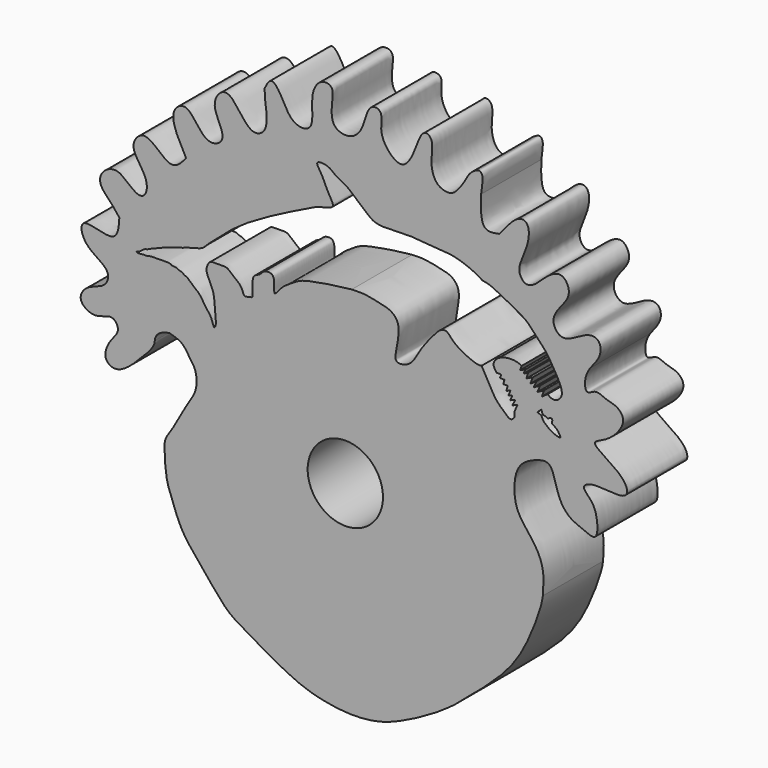
from build123d import *

# Parameters (mm, degrees)
F1_DEPTH  = 6.35
F3_DEPTH  = 25.4
F5_DEPTH  = 25.4
F6_R      = 3.175
F7_DEPTH  = 25.4
F8_DEPTH  = 6.35
F10_DEPTH = 25.4


with BuildPart() as f1:
    # F0 (on Front) → F1 (new body)
    with BuildSketch(Plane.XZ):
        with BuildLine():
            add(Edge.make_bspline(
                [(10.9984036535, 24.0315832198), (11.2508201386, 23.8778308248), (11.5032366237, 23.7240784298), (11.5215126425, 23.4777014703)],
                knots=[0, 0, 0, 0, 0.0447233475, 0.0447233475, 0.0447233475, 0.0447233475], degree=3))
            add(Edge.make_bspline(
                [(10.9984036535, 24.0315832198), (11.318751732, 24.2589387251), (11.9002035172, 24.6716031777), (12.4772696509, 24.5492373746), (12.7513167847, 24.476788925)],
                knots=[0, 0, 0, 0, 0.0600549328, 0.1090034566, 0.1090034566, 0.1090034566, 0.1090034566], degree=3))
            add(Edge.make_bspline(
                [(12.7513167847, 24.476788925), (12.7801536971, 24.4691654569), (13.1432187191, 24.3713046181), (13.9041914038, 24.1543272236), (14.4865013027, 23.118412087), (15.0212391704, 22.4815104313), (15.1483784966, 20.9912222479), (14.3534367186, 19.8288905944), (13.7773894226, 18.8194596912), (13.1463892826, 17.6016964054), (12.3275103111, 16.5516353367), (12.33673354, 15.5224584087), (12.4614385645, 13.4803711032), (12.9391618875, 12.3662133846), (13.3935402384, 11.0178879135), (13.885287327, 10.0483936843), (14.2166576245, 9.5778162211), (14.3705829978, 9.3592274934)],
                knots=[0.1090034566, 0.1090034566, 0.1090034566, 0.1090034566, 0.1141541191, 0.1734825658, 0.2342293124, 0.2866985313, 0.3540034981, 0.4216578627, 0.4838023186, 0.5515034671, 0.6159797954, 0.6739052407, 0.7551671162, 0.8199016797, 0.887742666, 0.9478551573, 1, 1, 1, 1], degree=3))
            add(Edge.make_bspline(
                [(14.3705829978, 9.3592274934), (14.7206651853, 8.9162577102), (15.4412953386, 8.0044221636), (16.7099442924, 6.5073513391), (17.7815135431, 5.221403597), (19.802190403, 4.1080383003), (22.0570488159, 2.7795203295), (24.6499909887, 1.5346825958), (28.0004167304, 1.0133030815), (30.4911131278, 1.2899704351), (32.5358810979, 2.0983522438), (35.0221117989, 3.4149839779), (36.2013376915, 4.264379538), (36.7506444454, 4.6600447968)],
                knots=[0, 0, 0, 0, 0.0782058444, 0.1609835967, 0.2374772319, 0.3265742131, 0.4230092715, 0.5241503873, 0.6331121598, 0.7261758396, 0.8140180236, 0.9133659154, 1, 1, 1, 1], degree=3))
            add(Edge.make_bspline(
                [(36.7506444454, 4.6600447968), (38.0482118698, 5.7380044032), (40.4681398718, 7.7483697897), (42.6588108138, 10.3810181384), (44.0911971273, 14.1984339335), (44.2071973729, 14.954150476), (44.2453101277, 15.2024468407)],
                knots=[0, 0, 0, 0, 0.3118653648, 0.5816204345, 0.8625382411, 1, 1, 1, 1], degree=3))
            add(Edge.make_bspline(
                [(44.2453101277, 15.2024468407), (44.2938227776, 15.848400886), (44.3896532958, 17.1244002587), (43.6653685125, 18.8179219808), (42.1824281003, 20.4121601043), (41.7448299587, 22.0053036238), (41.9549170872, 24.3004416385), (43.5573707454, 25.1201218431), (44.8828418523, 25.4189210069), (45.2842380478, 24.0145128143), (45.7035890114, 22.5708511362), (46.5789159349, 21.6207741355), (47.6415206601, 21.2667344741), (48.8901196768, 20.6378885116), (48.8646803505, 22.5006482664), (48.45281122, 23.5890104482), (47.4324727249, 24.3843013724), (48.2991800009, 24.9299049673), (49.7655119556, 24.745912619), (51.4805558413, 24.7166370614), (51.2824255696, 26.0405470322), (49.613217734, 27.141164769), (48.2215617536, 28.0385485724), (49.6100830633, 28.4546279683), (50.7055587208, 29.4428489996), (51.203797615, 30.5543020473), (50.4972683382, 31.3694856565), (49.523918889, 31.4773590202), (48.7198259044, 32.0094415516), (47.8360516345, 31.2174357433), (47.7324347795, 32.5701272714), (48.0509651737, 33.1047449245), (48.2145175338, 33.3792492747)],
                knots=[0, 0, 0, 0, 0.040744066, 0.0804846769, 0.1234849874, 0.1615884455, 0.2044023143, 0.2429972637, 0.2738845866, 0.3065024407, 0.3436012027, 0.3761355316, 0.4085263524, 0.4373910774, 0.4719923049, 0.5062540019, 0.5354026429, 0.5590121233, 0.5967931375, 0.6319390032, 0.6593392118, 0.7029962174, 0.7347840934, 0.7637562386, 0.8011345948, 0.8317135686, 0.8595523187, 0.8888743382, 0.9167130857, 0.9421066461, 0.9702741251, 1, 1, 1, 1], degree=3))
            add(Edge.make_bspline(
                [(48.2145175338, 33.3792492747), (48.5950355002, 33.8439156617), (49.2587706884, 34.6544304313), (49.0258880789, 35.8281927213), (47.8540536179, 35.9750774666), (45.8946501082, 34.3557167277), (44.8208041616, 35.9630519047), (45.7909681384, 37.2143462577), (46.7270923619, 38.3660487916), (45.9004450462, 39.8804900002), (44.462754299, 39.0181229163), (43.6562779713, 38.05713357), (42.7278190322, 37.7260580899), (42.1458451865, 38.5754480959), (42.3827930851, 39.4928006532), (42.9237980131, 40.5832499857), (43.1672501036, 41.9085122108), (42.8104534524, 42.6456809415), (41.9271647427, 42.5728848132), (41.1081073815, 41.5433021848), (40.5772328377, 40.8759750426)],
                knots=[0, 0, 0, 0, 0.0649588079, 0.1133072558, 0.162889424, 0.2379143585, 0.2939815841, 0.355441398, 0.4157416364, 0.4709310898, 0.5298717766, 0.5887591138, 0.6338079166, 0.679457886, 0.7275283161, 0.7843150664, 0.8428561205, 0.8840239325, 0.9248297557, 1, 1, 1, 1], degree=3))
            add(Edge.make_bspline(
                [(39.0425574679, 43.3239779902), (39.041356185, 43.2750910809), (39.0219364766, 42.5343034751), (38.9455255975, 40.5484904636), (40.0875605821, 40.77769754), (40.5772328377, 40.8759750426)],
                knots=[0.922393852, 0.922393852, 0.922393852, 0.922393852, 0.9255178455, 0.9680641617, 1, 1, 1, 1], degree=3))
            add(Edge.make_bspline(
                [(37.5906317725, 43.7307091179), (37.837040982, 44.0878360909), (38.2680272592, 44.6707408411), (38.9849891485, 45.0931421059), (39.0542753062, 44.2835962885), (39.0533749724, 43.7642026309), (39.0425574679, 43.3239779902)],
                knots=[0.8216596087, 0.8216596087, 0.8216596087, 0.8216596087, 0.8509906652, 0.8729404344, 0.8942624168, 0.922393852, 0.922393852, 0.922393852, 0.922393852], degree=3))
            add(Edge.make_bspline(
                [(20.7812990993, 45.2349446714), (20.9598079298, 45.5940884592), (21.3279572872, 46.3347720119), (22.249821537, 45.1800137174), (22.9935969334, 43.2743045581), (25.1488502819, 43.2665919302), (24.5153462292, 46.05875701), (25.4553091101, 47.4888604199), (26.6873108255, 47.2876915045), (26.3981434507, 45.832663308), (26.4326586416, 44.1475738694), (28.033955093, 43.8270222859), (29.0048714578, 44.7100760367), (29.2810737014, 45.9686995054), (29.7673820709, 47.0106125091), (30.7919294346, 46.7608773347), (30.4737375786, 45.4274062089), (30.9768926389, 44.0748322152), (32.5368669527, 42.8415889335), (33.5078035863, 44.7935011377), (33.9248822803, 46.1667164525), (34.4543244348, 46.441199242), (34.9775884722, 46.0257106289), (34.8859088958, 44.9334895069), (34.8042115189, 44.1708427609), (35.1252581337, 42.7624795784), (36.6346449921, 42.3082232141), (37.2318305413, 43.2058580932), (37.5522842498, 43.6751311032), (37.5906317725, 43.7307091179)],
                knots=[0, 0, 0, 0, 0.0277218275, 0.0571723705, 0.0983426517, 0.1308747904, 0.1751695472, 0.2104503073, 0.2359276255, 0.2684453241, 0.3038767035, 0.3359700253, 0.3670382979, 0.3999783047, 0.4285856537, 0.4517548965, 0.482396946, 0.5175640575, 0.5519099854, 0.5898501594, 0.6248167325, 0.6437016849, 0.6642895518, 0.6932428536, 0.7192839991, 0.751939533, 0.7835122944, 0.8170949524, 0.8216596087, 0.8216596087, 0.8216596087, 0.8216596087], degree=3))
            add(Edge.make_bspline(
                [(14.1616091132, 37.9098691046), (13.5322036704, 39.0585651197), (12.5165881256, 40.9121136432), (14.415081949, 42.2942809419), (15.6801738753, 39.2181703105), (17.8891113724, 40.288290195), (16.1164787578, 42.4584838578), (17.1043617929, 43.9976160978), (18.2133555313, 43.7714508614), (19.5101751542, 41.2574608503), (21.2098070485, 42.0889312218), (20.7967934332, 44.364971779), (20.7856516925, 44.9905561021), (20.7812990993, 45.2349446714)],
                knots=[0, 0, 0, 0, 0.1255875684, 0.2026494815, 0.3148208465, 0.394753195, 0.4994852093, 0.581932278, 0.6470220286, 0.7573364877, 0.8326463523, 0.9346222132, 1, 1, 1, 1], degree=3))
            add(Edge.make_bspline(
                [(8.5367122665, 31.6628292203), (8.3127892358, 31.9583180313), (7.8541426883, 32.563547974), (6.8806160847, 33.4557075972), (6.8883368651, 34.3315498499), (7.47477818, 34.9861300171), (8.3402060898, 35.1611632264), (8.970020513, 34.7214135391), (9.6560863557, 34.1403407566), (10.1718011229, 33.8172376038), (10.7815639847, 33.9576662574), (10.978297702, 35.0741741128), (10.2142510997, 36.2695531421), (9.4105325611, 37.4621624953), (10.7801226417, 39.1527841943), (12.8559031413, 36.3266719936), (13.7632400269, 37.4268378556), (14.1616091132, 37.9098691046)],
                knots=[0, 0, 0, 0, 0.0694766566, 0.1423043829, 0.198764402, 0.2572227337, 0.3150056147, 0.3706419002, 0.4324868971, 0.4819124791, 0.5268043346, 0.5899069271, 0.6677982109, 0.7421643789, 0.816159908, 0.9192844349, 1, 1, 1, 1], degree=3))
            add(Edge.make_bspline(
                [(11.5215126425, 23.4777014703), (11.5519824112, 23.0669419365), (10.2609372621, 21.6762525704), (8.4228613972, 19.9629948924), (7.0758637078, 20.791261283), (7.7048728638, 22.3612173674), (8.6771579986, 23.1802967965), (7.9435187696, 24.4141861888), (6.5366962855, 23.4032665751), (4.921446276, 24.3963742293), (5.7309585025, 25.8129083909), (7.4360032754, 26.0087969672), (7.8559307485, 27.6450981333), (5.5063417726, 28.4696216823), (5.0165874684, 31.0102223234), (8.3946531142, 29.35366443), (8.4920119608, 30.9362278683), (8.5367122665, 31.6628292203)],
                knots=[0.0447233475, 0.0447233475, 0.0447233475, 0.0447233475, 0.1192860883, 0.1999034705, 0.251345599, 0.3134883632, 0.3693216082, 0.417594106, 0.4791297169, 0.5399528379, 0.5960189727, 0.661036052, 0.7147344751, 0.7926602543, 0.8538783164, 0.9329112437, 1, 1, 1, 1], degree=3))
        make_face()
        with BuildLine():
            add(Edge.make_bspline(
                [(37.5906317725, 43.7307091179), (37.6583476274, 43.8577441648), (37.7894200704, 44.1020132691), (37.9701475696, 44.4125750304), (38.2660625267, 44.7503024581), (38.617932892, 44.9570790944), (38.9662554933, 45.071039684), (39.1943363106, 44.7057833587), (39.1494306301, 44.1431294325), (39.0811155736, 43.6150886764), (39.0425574679, 43.3239779902)],
                knots=[0, 0, 0, 0, 0.1208224911, 0.2327121383, 0.3564976038, 0.4773631849, 0.5804917461, 0.6891217609, 0.828579593, 1, 1, 1, 1], degree=3))
            add(Edge.make_bspline(
                [(37.5906317725, 43.7307091179), (37.837040982, 44.0878360909), (38.2680272592, 44.6707408411), (38.9849891485, 45.0931421059), (39.0542753062, 44.2835962885), (39.0533749724, 43.7642026309), (39.0425574679, 43.3239779902)],
                knots=[0.8216596087, 0.8216596087, 0.8216596087, 0.8216596087, 0.8509906652, 0.8729404344, 0.8942624168, 0.922393852, 0.922393852, 0.922393852, 0.922393852], degree=3))
        make_face()
    extrude(amount=F1_DEPTH)

    # F2 (on face) → F3 (cut)
    with BuildSketch(Plane.XZ.offset(6.35)):
        with BuildLine():
            add(Edge.make_bspline(
                [(10.9213702381, 30.0800928582), (11.0621325147, 30.1711970051), (11.4478540925, 30.3014983827), (12.6817518677, 30.859944003), (13.7072983183, 31.0710903888), (14.3208772689, 31.3579432612), (15.564229897, 31.570259495), (16.0136899008, 32.1813542456), (17.049722233, 32.9854347042), (18.3746171419, 34.2826629705), (21.6392706703, 36.1544500181), (23.5400043531, 37.0799669008), (24.4557429105, 37.5258624554)],
                knots=[0, 0, 0, 0, 0.0624681448, 0.1605025237, 0.2463917171, 0.3163794584, 0.4075323766, 0.479568724, 0.5724130102, 0.6875313423, 0.8499041867, 1, 1, 1, 1], degree=3))
            add(Edge.make_bspline(
                [(10.9213702381, 30.0800928582), (10.8182955843, 30.060403049), (10.6160561956, 30.0217703219), (10.4055464041, 29.8084417721), (10.1990968304, 29.6832850534), (9.8446723952, 29.5882293745), (10.2918300979, 29.5188273702), (10.5647671852, 29.602504464), (10.8901845547, 29.5492359826), (11.1801832433, 29.6758527354), (11.4710576538, 29.6348812436), (11.8361269725, 29.6727692435), (12.0701749285, 29.6638357746), (12.3013535347, 29.6671041387), (12.4604577777, 29.6625090516), (12.642664173, 29.6801227261), (12.9175606543, 29.6119395683), (12.9813179246, 29.5210420262), (13.2639078187, 29.5491884683), (13.4567806443, 29.4620166023), (13.6101856596, 29.3803257023), (13.8016463931, 29.3527375965), (13.9617442467, 29.2057757716), (14.262979255, 29.0863052722), (14.33562829, 29.011155294), (14.5563019527, 28.8115816148), (14.7331123665, 28.6495022445), (14.9650783705, 28.4431672158), (15.2472798972, 28.2700092196), (15.6300765823, 27.7063340855), (15.9140629032, 27.229935805), (16.3288629431, 26.8078143592), (16.4898288734, 25.9640936837), (16.7113330192, 26.3395278682), (16.6440586968, 26.8944387045), (16.6245707773, 27.4260731323), (16.5646216855, 27.9561127995), (16.4922967389, 28.7242841841), (16.2171922513, 29.228497163), (16.0502440225, 29.60383452), (15.8498940382, 30.0972798293), (15.9242114176, 30.4715311828), (16.1301596613, 30.8951597944), (16.5022073659, 30.9337885236), (16.8598977355, 30.925444839), (17.2230428243, 30.9204375143), (17.6123193522, 30.9510625485), (18.0208450694, 30.5484633884), (18.4124488922, 30.2275658458), (18.8579724683, 29.9205017207), (19.0273748777, 29.2065876594), (19.2289940195, 29.3060397701), (19.3648556717, 29.2536751868), (19.5658344037, 29.4027199569), (19.6758211775, 29.3466416068), (19.7907481863, 29.4687530524), (19.7426666547, 29.679034281), (19.7359344634, 30.6677243546), (19.9019423697, 31.1236509256), (20.4493921261, 31.280142146), (20.6617274484, 31.6822365954), (21.4582760395, 31.7883774062), (21.6455719921, 31.155598957), (21.5160445037, 29.953434889), (22.1189328434, 30.89800932), (22.8009179427, 31.3425690523), (23.5862555743, 31.8845985236), (24.3790029645, 32.1394947537), (25.5496803949, 32.34015209), (26.4432119532, 32.5062561098), (27.304817882, 32.5973834381), (27.8581011731, 32.6687042567), (28.1333383173, 32.7041836191)],
                knots=[0, 0, 0, 0, 0.0124943974, 0.0245148463, 0.0364334491, 0.0467508795, 0.058726404, 0.0716998514, 0.0842925533, 0.0966964264, 0.1089343296, 0.1225436985, 0.1336494248, 0.144351145, 0.1532555432, 0.163099707, 0.1747943426, 0.1819615768, 0.1934698517, 0.2040261437, 0.2133410066, 0.2229314519, 0.2336489854, 0.2462026284, 0.2537133066, 0.2656888042, 0.277132901, 0.289381368, 0.3023902215, 0.3208309997, 0.3377388974, 0.3559011538, 0.3738992488, 0.3842692937, 0.4015763024, 0.418119285, 0.4346836826, 0.454495423, 0.4714671739, 0.4860581943, 0.5021549002, 0.5161409215, 0.5308917231, 0.5440478608, 0.5576495421, 0.5712512234, 0.5848836089, 0.6015159078, 0.6177276563, 0.6346555721, 0.6524091162, 0.6608042319, 0.6691994042, 0.6799011415, 0.6871715086, 0.6950641937, 0.7053460917, 0.7277566769, 0.7432686553, 0.7591566332, 0.7741434845, 0.7919830937, 0.8097539618, 0.8299061546, 0.8480781119, 0.8698967765, 0.8915050665, 0.9122189323, 0.9367396177, 0.958502005, 0.9793563445, 1, 1, 1, 1], degree=3))
            add(Edge.make_bspline(
                [(28.1333383173, 32.7041836191), (28.4447338183, 32.7147448415), (29.1283937094, 32.760138923), (30.4928781187, 32.4625611087), (31.4747994534, 32.2455623678), (32.1565235724, 31.4999370771), (32.059282622, 30.2460859406), (31.8173684326, 29.1896037218), (31.792310072, 28.5462210928), (32.4201594265, 28.4647743828), (33.1831286949, 28.8241096157), (33.5558384411, 29.5009799351), (34.0187523078, 30.2669265073), (34.5293868658, 30.9637754806), (35.1225494167, 31.6599302024), (35.5084483018, 32.0909391799), (36.1265305642, 32.3579699138), (36.6667314638, 31.5645481621), (37.6564672856, 30.9817736061), (38.6799457652, 30.5513126095), (38.973828395, 30.5873574143), (39.0821322799, 30.6006409228)],
                knots=[0, 0, 0, 0, 0.0569144606, 0.1245771675, 0.1817876373, 0.2355106649, 0.2987629217, 0.359895433, 0.4006617079, 0.4408969185, 0.4925680808, 0.542591235, 0.5965146494, 0.6504445858, 0.7049104477, 0.7489486043, 0.7902974011, 0.8423332006, 0.9057877046, 0.965265946, 1, 1, 1, 1], degree=3))
            add(Edge.make_bspline(
                [(39.0821322799, 30.6006409228), (39.2965137066, 30.2458058271), (39.7205354547, 29.5441861059), (40.218174815, 28.4578704854), (41.0526669064, 27.7505771838), (41.5272187519, 27.2917509414), (42.0679852633, 27.8149798012), (41.4297583603, 28.9211768264), (40.8534983099, 30.056962233), (39.8275546559, 30.9348100284), (40.5191768137, 31.8051609064), (41.7155009482, 31.9744597758), (42.5513788626, 31.7177248026), (43.7825538999, 30.8855475191), (44.5622137989, 30.3708020434), (45.1623077351, 29.8853459199), (46.2152371998, 30.5913010892), (45.1848802623, 32.3130075341), (44.5962190379, 33.3763475906), (43.6647534314, 34.2907294849), (43.0457859768, 35.0790449938), (41.9609214475, 35.7636010234), (40.9091454733, 36.2240410817), (39.9405635142, 36.8174269381), (39.3920691489, 36.9128081003), (39.140265435, 36.9565971196)],
                knots=[0, 0, 0, 0, 0.0471289622, 0.0934992279, 0.1381013781, 0.1691653891, 0.1983013447, 0.2437746361, 0.2940659419, 0.3389748368, 0.3774362068, 0.4229118573, 0.4627941098, 0.5140815647, 0.5559837663, 0.5903984763, 0.62926846, 0.6853848868, 0.734378372, 0.7815503832, 0.8241503815, 0.8714534974, 0.917581552, 0.9622845444, 1, 1, 1, 1], degree=3))
            add(Edge.make_bspline(
                [(24.4557429105, 37.5258624554), (24.7253385406, 37.6679074084), (25.269000354, 37.9543527664), (26.2041876384, 38.1068656578), (26.7222447476, 38.390498104), (26.0571499962, 39.2934646114), (25.7120527401, 40.3463293225), (25.0259646789, 41.1902198608), (25.6192781851, 41.3211522067), (26.2749340242, 41.1753665803), (26.7558685385, 40.6898514014), (27.5394779114, 40.37141568), (28.333800935, 39.7426144748), (29.3119296607, 38.8398867041), (29.9261777829, 38.3487917662), (30.5795011701, 38.2059401352), (31.5837794212, 38.2066358352), (32.438061969, 38.2621120222), (33.4591861971, 38.2772266445), (34.2594025193, 38.1616941856), (35.5273603681, 38.1006369361), (36.9245225402, 38.0116693913), (38.5905711621, 37.3317489081), (38.9903120203, 37.0589363552), (39.140265435, 36.9565971196)],
                knots=[0, 0, 0, 0, 0.0462405859, 0.0932479536, 0.12352938, 0.1694573257, 0.2239012849, 0.2673722591, 0.2966816534, 0.3360973889, 0.3752190307, 0.4184715797, 0.4672989686, 0.5228690875, 0.5647361691, 0.6030394988, 0.6506723572, 0.6959270297, 0.7435553104, 0.786874903, 0.8398639848, 0.8982460293, 0.9618293826, 1, 1, 1, 1], degree=3))
        make_face()
    extrude(amount=-F3_DEPTH, mode=Mode.SUBTRACT)

    # F4 (on face) → F5 (cut)
    with BuildSketch(Plane.XZ.offset(6.35)):
        with BuildLine():
            Line((41.6713940372, 29.2312545242), (41.334032409, 29.1238261514))
            add(Edge.make_bspline(
                [(41.4966993879, 28.8241959522), (41.4898705966, 28.8366803131), (41.4346962394, 28.9376267554), (41.3810155374, 29.0374196072), (41.334032409, 29.1238261514)],
                knots=[0.2423069379, 0.2423069379, 0.2423069379, 0.2423069379, 0.2437746361, 0.2541872492, 0.2541872492, 0.2541872492, 0.2541872492], degree=3))
            Line((41.4966993879, 28.8241959522), (41.6713940372, 29.2312545242))
        make_face()
        with BuildLine():
            Line((41.5145814011, 29.5445260139), (41.1690312073, 29.4201169181))
            add(Edge.make_bspline(
                [(41.334032409, 29.1238261514), (41.2795068463, 29.2241039661), (41.2250699584, 29.3229570106), (41.1690312073, 29.4201169181)],
                knots=[0.2541872492, 0.2541872492, 0.2541872492, 0.2541872492, 0.2662714507, 0.2662714507, 0.2662714507, 0.2662714507], degree=3))
            Line((41.334032409, 29.1238261514), (41.5145814011, 29.5445260139))
        make_face()
        with BuildLine():
            Line((41.286166143, 29.8312112658), (40.9100426519, 29.8312112658))
            add(Edge.make_bspline(
                [(41.1690312073, 29.4201169181), (41.0877859462, 29.560979837), (41.0031736736, 29.6982838928), (40.9100426519, 29.8312112658)],
                knots=[0.2662714507, 0.2662714507, 0.2662714507, 0.2662714507, 0.2837911864, 0.2837911864, 0.2837911864, 0.2837911864], degree=3))
            Line((41.1690312073, 29.4201169181), (41.286166143, 29.8312112658))
        make_face()
        with BuildLine():
            Line((41.0126723506, 30.1930415904), (40.6225825999, 30.1930415904))
            add(Edge.make_bspline(
                [(40.9100426519, 29.8312112658), (40.855424335, 29.9091688492), (40.7634152709, 30.0314018438), (40.6612602523, 30.1493652065), (40.6225825999, 30.1930415904)],
                knots=[0.2837911864, 0.2837911864, 0.2837911864, 0.2837911864, 0.2940659419, 0.3002186185, 0.3002186185, 0.3002186185, 0.3002186185], degree=3))
            Line((40.9100426519, 29.8312112658), (41.0126723506, 30.1930415904))
        make_face()
        with BuildLine():
            Line((40.7454008838, 30.4925257189), (40.3571343923, 30.4925257189))
            add(Edge.make_bspline(
                [(40.6225825999, 30.1930415904), (40.5320847441, 30.2952354632), (40.439304801, 30.3946633916), (40.3571343923, 30.4925257189)],
                knots=[0.3002186185, 0.3002186185, 0.3002186185, 0.3002186185, 0.314614633, 0.314614633, 0.314614633, 0.314614633], degree=3))
            Line((40.6225825999, 30.1930415904), (40.7454008838, 30.4925257189))
        make_face()
        with BuildLine():
            Line((41.9159745094, 28.9785182312), (41.4966993879, 28.8241959522))
            add(Edge.make_bspline(
                [(41.6710244801, 28.4980648038), (41.616475288, 28.6059420617), (41.5561130832, 28.7155761421), (41.4966993879, 28.8241959522)],
                knots=[0.2295372734, 0.2295372734, 0.2295372734, 0.2295372734, 0.2423069379, 0.2423069379, 0.2423069379, 0.2423069379], degree=3))
            Line((41.6710244801, 28.4980648038), (41.9159745094, 28.9785182312))
        make_face()
        with BuildLine():
            Line((42.1091548788, 28.6834057337), (41.6710244801, 28.4980648038))
            add(Edge.make_bspline(
                [(41.8422915446, 28.0821289639), (41.8062706466, 28.2132539764), (41.7438242883, 28.354094868), (41.6710244801, 28.4980648038)],
                knots=[0.2124952405, 0.2124952405, 0.2124952405, 0.2124952405, 0.2295372734, 0.2295372734, 0.2295372734, 0.2295372734], degree=3))
            Line((41.8422915446, 28.0821289639), (42.1091548788, 28.6834057337))
        make_face()
        with BuildLine():
            add(Edge.make_bspline(
                [(44.3582837297, 30.4997689852), (44.4374421462, 30.4447879408), (44.5327238499, 30.3770619111), (44.6247899032, 30.30869081), (44.6434171224, 30.2949218932)],
                knots=[0.5428271829, 0.5428271829, 0.5428271829, 0.5428271829, 0.5559837663, 0.5593379184, 0.5593379184, 0.5593379184, 0.5593379184], degree=3))
            Line((44.3582837297, 30.4997689852), (44.1494948367, 29.9524613109))
            Line((44.1494948367, 29.9524613109), (44.6434171224, 30.2949218932))
        make_face()
        with BuildLine():
            add(Edge.make_bspline(
                [(44.0159770479, 30.7322263029), (44.1379794371, 30.650526509), (44.2510957097, 30.5742185452), (44.3582837297, 30.4997689852)],
                knots=[0.5250119184, 0.5250119184, 0.5250119184, 0.5250119184, 0.5428271829, 0.5428271829, 0.5428271829, 0.5428271829], degree=3))
            Line((44.0159770479, 30.7322263029), (43.7830370587, 30.1744778601))
            Line((43.7830370587, 30.1744778601), (44.3582837297, 30.4997689852))
        make_face()
        with BuildLine():
            add(Edge.make_bspline(
                [(43.7000024975, 30.9435123), (43.7272811413, 30.9252565127), (43.8377239446, 30.8513166481), (43.9411238646, 30.7823522857), (44.0159770479, 30.7322263029)],
                knots=[0.5105589264, 0.5105589264, 0.5105589264, 0.5105589264, 0.5140815647, 0.5250119184, 0.5250119184, 0.5250119184, 0.5250119184], degree=3))
            Line((43.7000024975, 30.9435123), (43.4753444355, 30.4215302703))
            Line((43.4753444355, 30.4215302703), (44.0159770479, 30.7322263029))
        make_face()
        with BuildLine():
            add(Edge.make_bspline(
                [(43.3967219254, 31.1452016194), (43.5006472148, 31.076841158), (43.602620942, 31.0086833173), (43.7000024975, 30.9435123)],
                knots=[0.497983521, 0.497983521, 0.497983521, 0.497983521, 0.5105589264, 0.5105589264, 0.5105589264, 0.5105589264], degree=3))
            Line((43.3967219254, 31.1452016194), (43.186634779, 30.6006409228))
            Line((43.186634779, 30.6006409228), (43.7000024975, 30.9435123))
        make_face()
        with BuildLine():
            add(Edge.make_bspline(
                [(43.0220411563, 31.3853100285), (43.1467333504, 31.3081107617), (43.2731081606, 31.2265128579), (43.3967219254, 31.1452016194)],
                knots=[0.4830257258, 0.4830257258, 0.4830257258, 0.4830257258, 0.497983521, 0.497983521, 0.497983521, 0.497983521], degree=3))
            Line((43.0220411563, 31.3853100285), (42.8539392565, 30.8837774003))
            Line((42.8539392565, 30.8837774003), (43.3967219254, 31.1452016194))
        make_face()
        with BuildLine():
            add(Edge.make_bspline(
                [(42.7754646929, 31.5328878026), (42.8560183336, 31.4865965745), (42.9386534918, 31.4369368895), (43.0220411563, 31.3853100285)],
                knots=[0.4730227291, 0.4730227291, 0.4730227291, 0.4730227291, 0.4830257258, 0.4830257258, 0.4830257258, 0.4830257258], degree=3))
            Line((42.7754646929, 31.5328878026), (42.6227713228, 31.1592284084))
            Line((42.6227713228, 31.1592284084), (43.0220411563, 31.3853100285))
        make_face()
        with BuildLine():
            add(Edge.make_bspline(
                [(42.4665844344, 31.6972087628), (42.4895232501, 31.6862187151), (42.5882332405, 31.6375128271), (42.6930941251, 31.5802231521), (42.7754646929, 31.5328878026)],
                knots=[0.4596479026, 0.4596479026, 0.4596479026, 0.4596479026, 0.4627941098, 0.4730227291, 0.4730227291, 0.4730227291, 0.4730227291], degree=3))
            Line((42.4665844344, 31.6972087628), (42.3225612666, 31.3194634379))
            Line((42.3225612666, 31.3194634379), (42.7754646929, 31.5328878026))
        make_face()
    extrude(amount=-F5_DEPTH, mode=Mode.SUBTRACT)

    # F6 (on face) → F7 (cut)
    with BuildSketch(Plane.XZ.offset(6.35)):
        with Locations((27.5912359357, 18.1433614343)):
            Circle(F6_R)
    extrude(amount=-F7_DEPTH, mode=Mode.SUBTRACT)

    # F0 (on Front) → F8 (join)
    with BuildSketch(Plane.XZ):
        with BuildLine():
            add(Edge.make_bspline(
                [(10.9984036535, 24.0315832198), (11.318751732, 24.2589387251), (11.9002035172, 24.6716031777), (12.4772696509, 24.5492373746), (12.7513167847, 24.476788925)],
                knots=[0, 0, 0, 0, 0.0600549328, 0.1090034566, 0.1090034566, 0.1090034566, 0.1090034566], degree=3))
            add(Edge.make_bspline(
                [(10.9984036535, 24.0315832198), (11.2508201386, 23.8778308248), (11.5032366237, 23.7240784298), (11.5215126425, 23.4777014703)],
                knots=[0, 0, 0, 0, 0.0447233475, 0.0447233475, 0.0447233475, 0.0447233475], degree=3))
            add(Edge.make_bspline(
                [(11.5215126425, 23.4777014703), (11.5392012744, 23.5946353064), (11.5756340739, 23.8354705957), (11.8455379568, 24.1597099761), (12.2184574101, 24.3495145074), (12.5653452639, 24.432595118), (12.7513167847, 24.476788925)],
                knots=[0, 0, 0, 0, 0.2280423509, 0.4696427557, 0.715624518, 1, 1, 1, 1], degree=3))
        make_face()
    extrude(amount=F8_DEPTH)

    # F9 (on face) → F10 (cut)
    with BuildSketch(Plane.XZ.offset(6.35)):
        with BuildLine():
            Line((44.2335531116, 28.6649558693), (44.1137738526, 28.9916228503))
            Line((44.1137738526, 28.9916228503), (43.7871105969, 28.6867339164))
            Line((43.7871105969, 28.6867339164), (44.1137738526, 28.5560674965))
            add(Edge.make_bspline(
                [(44.1137738526, 28.5560674965), (44.1652612256, 28.4297421428), (44.2631035792, 28.1896838679), (44.520164761, 27.9924948641), (44.8164936061, 27.7279458062), (45.1788694335, 27.5229034658), (45.8299014386, 27.3226379438), (45.6008222005, 27.7340944328), (45.4113728546, 28.0000007739), (45.1377270972, 28.1482587535), (45.0098581466, 28.2332774706)],
                knots=[0, 0, 0, 0, 0.0986624584, 0.1874899919, 0.2848353168, 0.3946153172, 0.5037034412, 0.5866683488, 0.6840135227, 0.7820097536, 0.7820097536, 0.7820097536, 0.7820097536], degree=3))
            add(Edge.make_bspline(
                [(45.0098581466, 28.2332774706), (44.9903732387, 28.2462327805), (44.8600896248, 28.3355105035), (44.7470482524, 28.4393734682), (44.6494537002, 28.5070783077)],
                knots=[0.7820097536, 0.7820097536, 0.7820097536, 0.7820097536, 0.7969426011, 0.8829889012, 0.8829889012, 0.8829889012, 0.8829889012], degree=3))
            add(Edge.make_bspline(
                [(44.6494537002, 28.5070783077), (44.6235136147, 28.5250738749), (44.4903395266, 28.6096255153), (44.3480395656, 28.6402872122), (44.2335531116, 28.6649558693)],
                knots=[0.8829889012, 0.8829889012, 0.8829889012, 0.8829889012, 0.905859526, 1, 1, 1, 1], degree=3))
        make_face()
        with BuildLine():
            add(Edge.make_bspline(
                [(44.6494537002, 28.5070783077), (44.7986195019, 28.5726133736), (45.0936628307, 28.6987699351), (45.0371072395, 28.3876168964), (45.0098581466, 28.2332774706)],
                knots=[0, 0, 0, 0, 0.503792919, 1, 1, 1, 1], degree=3))
            add(Edge.make_bspline(
                [(45.0098581466, 28.2332774706), (44.9903732387, 28.2462327805), (44.8600896248, 28.3355105035), (44.7470482524, 28.4393734682), (44.6494537002, 28.5070783077)],
                knots=[0.7820097536, 0.7820097536, 0.7820097536, 0.7820097536, 0.7969426011, 0.8829889012, 0.8829889012, 0.8829889012, 0.8829889012], degree=3))
        make_face()
    extrude(amount=-F10_DEPTH, mode=Mode.SUBTRACT)


solid = f1.part
